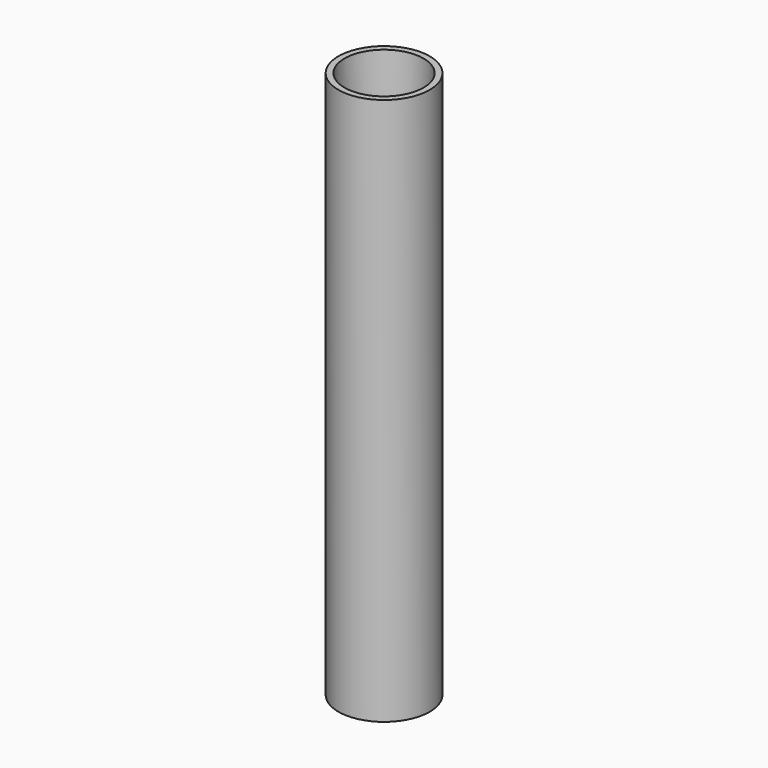
from build123d import *

# Parameters (mm, degrees)
F0_R     = 3.75
F1_DEPTH = 45
F2_R     = 3.25
F3_DEPTH = 22.5
F5_R     = 3.25
F6_DEPTH = 22.5
F7_SIZE2 = 0.49999
F7_SIZE  = 22.49999


# Not quite as in the source:
# - a fillet or chamfer that OpenCascade refuses, or shapes differently, is made with other operations: its cross-section is extruded or revolved along the edge and cut away or added
# - a fillet or chamfer is up to 0.001 mm smaller than in the source, because OpenCascade refuses the exact size


with BuildPart() as f1:
    # F0 (on Top) → F1 (new body)
    with BuildSketch(Plane.XY):
        Circle(F0_R)
    extrude(amount=F1_DEPTH)

    # F2 (on face) → F3 (cut)
    with BuildSketch(Plane.XY):
        Circle(F2_R)
    extrude(amount=F3_DEPTH, mode=Mode.SUBTRACT)

    # F4: chamfer of 25 x 0.5 on 1 edges, made by hand


with BuildPart() as f4_tool2:
    # F4_s3 → F4_t4 (revolve)
    with BuildSketch(Plane.XZ):
        Polygon((3.25, -2.5), (2.75, 22.5), (3.25, 22.5), align=None)
    revolve(axis=Axis((0, 0, 22.5), (0, 0, 1)))

    split(bisect_by=Plane.XY, keep=Keep.TOP)


with BuildPart() as f1_1:
    add(f1.part)

    # F4_t1: union F4_tool2
    add(f4_tool2.part)

    # F5 (on face) → F6 (cut)
    with BuildSketch(Plane.XY.offset(45)):
        Circle(F5_R)
    extrude(amount=-F6_DEPTH, mode=Mode.SUBTRACT)

    # F7 (size 22.5 and 0.5 in the source; OpenCascade refuses exactly that, so slightly less here)
    f7_edges = [f1_1.edges().sort_by_distance(p)[0] for p in [
        (-3.25, 0, 22.5),
    ]]
    f7_side = f1_1.faces().sort_by_distance((-3.25, 0, 33.75))[0]
    chamfer(f7_edges, length=F7_SIZE, length2=F7_SIZE2, reference=f7_side)


solid = f1_1.part
